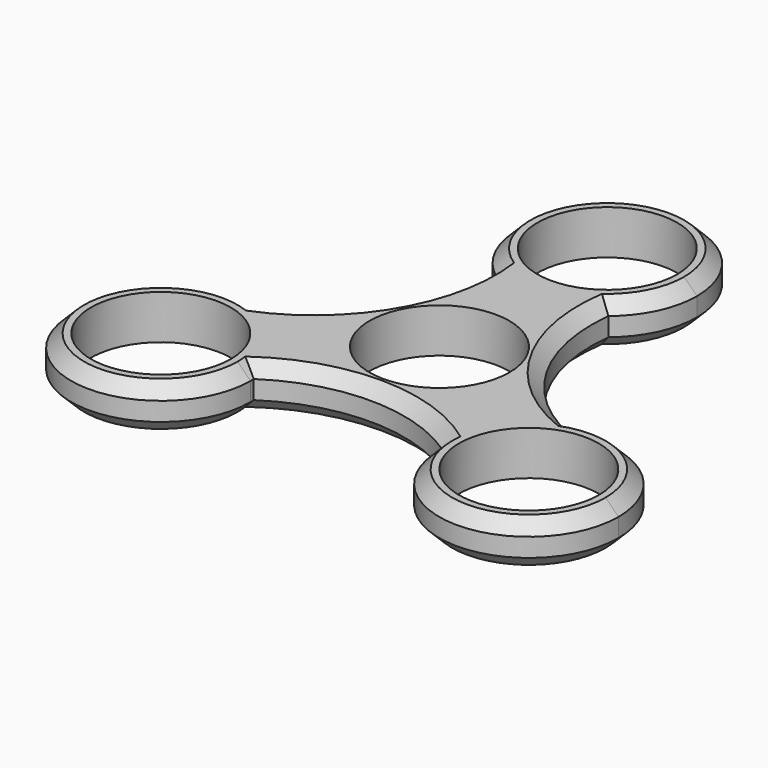
from build123d import *

# Parameters (mm, degrees)
F0_R     = 11.049
F0_R_2   = 11.05
F1_DEPTH = 7
F2_SIZE  = 2.032


# Not quite as in the source:
# - a feature names something its author has since deleted; it is built from what else it names


with BuildPart() as f1:
    # F0 (on Top) → F1 (new body)
    with BuildSketch(Plane.XY):
        with BuildLine():
            ThreePointArc((-8.7042735718, 22.0943097642), (-12.2328176499, 5.8189544339), (-24.7131356106, -5.2073540163))
            ThreePointArc((-24.7131356106, -5.2073540163), (-17.821671092, -10.084264276), (-14.930456808, -18.0163142542))
            ThreePointArc((-14.930456808, -18.0163142542), (0.0145480917, -13.5128951169), (14.9256967567, -18.1271773868))
            ThreePointArc((14.9256967567, -18.1271773868), (17.7880815001, -10.1284239204), (24.7131356106, -5.2073540163))
            ThreePointArc((24.7131356106, -5.2073540163), (12.1415366781, 5.9758444424), (8.7441728022, 22.4551328426))
            ThreePointArc((8.7441728022, 22.4551328426), (0.0821273079, 19.2679731194), (-8.7042735718, 22.0943097642))
        make_face()
        Circle(F0_R, mode=Mode.SUBTRACT)
        with BuildLine():
            ThreePointArc((-14.930456808, -18.0163142542), (-17.821671092, -10.084264276), (-24.7131356106, -5.2073540163))
            ThreePointArc((-24.7131356106, -5.2073540163), (-40.5273347614, -27.0082695647), (-14.9149335915, -18.6791807883))
            ThreePointArc((-14.9149335915, -18.6791807883), (-14.9188149276, -18.3476566518), (-14.930456808, -18.0163142542))
        make_face()
        with Locations((-29.0754335915, -18.6791807883)):
            Circle(F0_R_2, mode=Mode.SUBTRACT)
        with BuildLine():
            ThreePointArc((13.9525783408, 33.428221941), (-6.5471611927, 46.095014193), (-8.7042735718, 22.0943097642))
            ThreePointArc((-8.7042735718, 22.0943097642), (0.0821273079, 19.2679731194), (8.7441728022, 22.4551328426))
            ThreePointArc((8.7441728022, 22.4551328426), (12.5843929813, 27.3549984844), (13.9525783408, 33.428221941))
        make_face()
        with Locations((-0.2106978791, 33.428221941)):
            Circle(F0_R_2, mode=Mode.SUBTRACT)
        with BuildLine():
            ThreePointArc((24.7131356106, -5.2073540163), (17.7880815001, -10.1284239204), (14.9256967567, -18.1271773868))
            ThreePointArc((14.9256967567, -18.1271773868), (28.7993794297, -32.8369897413), (43.2359335915, -18.6791807883))
            ThreePointArc((43.2359335915, -18.6791807883), (37.404522368, -7.2272796184), (24.7131356106, -5.2073540163))
        make_face()
        with Locations((29.0754335915, -18.6791807883)):
            Circle(F0_R_2, mode=Mode.SUBTRACT)
    extrude(amount=F1_DEPTH)

    # F2
    f2_edges = [f1.edges().sort_by_distance(p)[0] for p in [
        (-12.232818, 5.818954, 7),
        (12.141537, 5.975844, 7),
        (0.014548, -13.512895, 7),
        (0.014548, -13.512895, 0),
        (12.141537, 5.975844, 0),
        (-12.232818, 5.818954, 0),
        (-40.329196, -27.274097, 0),
        (40.362786, -27.229938, 0),
        (-0.503523, 47.588471, 0),
        (-40.329196, -27.274097, 7),
        (40.362786, -27.229938, 7),
        (-0.503523, 47.588471, 7),
    ]]
    chamfer(f2_edges, length=F2_SIZE)


solid = f1.part
